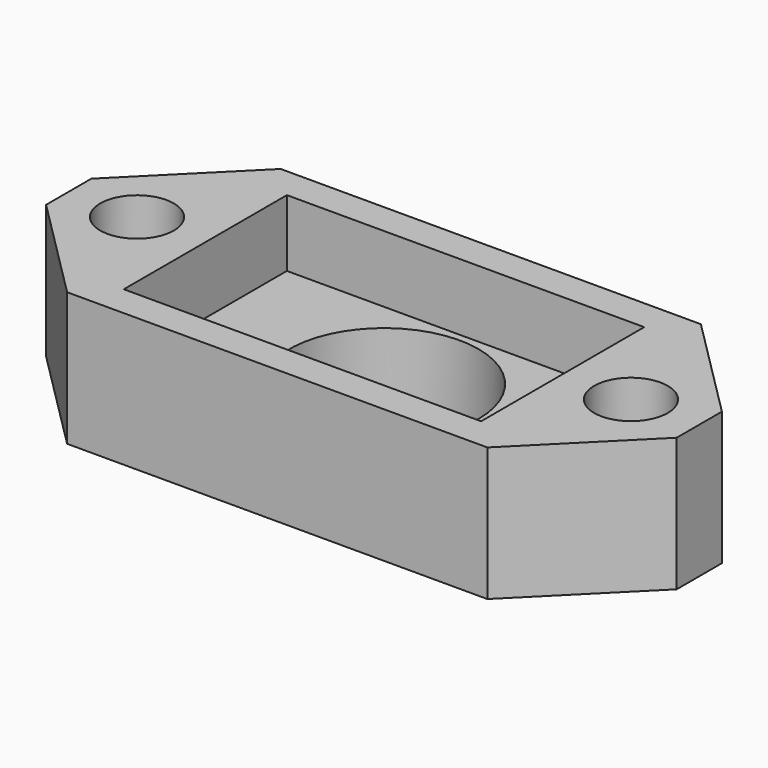
from build123d import *

# Parameters (mm, degrees)
F0_R     = 1.75
F0_W     = 17
F0_H     = 9.7
F1_DEPTH = 6.35
F0_R_2   = 4.5
F2_DEPTH = 3.175


# Not quite as in the source:
# - a length typed as a fraction of an inch, garbled in the dataset ("3 / 203.2 mm" for 3/8 in), is restored


with BuildPart() as f1:
    # F0 (on Top) → F1 (new body)
    with BuildSketch(Plane.XY):
        Polygon((9.9961940777, 6.35), (-9.9961940777, 6.35), (-15, 1.3461940777), (-15, -1.3461940777), (-9.9961940777, -6.35), (9.9961940777, -6.35), (15, -1.3461940777), (15, 1.3461940777), align=None)
        with Locations((-11.75, 0)):
            Circle(F0_R, mode=Mode.SUBTRACT)
        Rectangle(F0_W, F0_H, mode=Mode.SUBTRACT)
        with Locations((11.75, 0)):
            Circle(F0_R, mode=Mode.SUBTRACT)
    extrude(amount=F1_DEPTH)

    # F0 (on Top) → F2 (join)
    with BuildSketch(Plane.XY):
        Rectangle(F0_W, F0_H)
        Circle(F0_R_2, mode=Mode.SUBTRACT)
    extrude(amount=F2_DEPTH)


solid = f1.part
